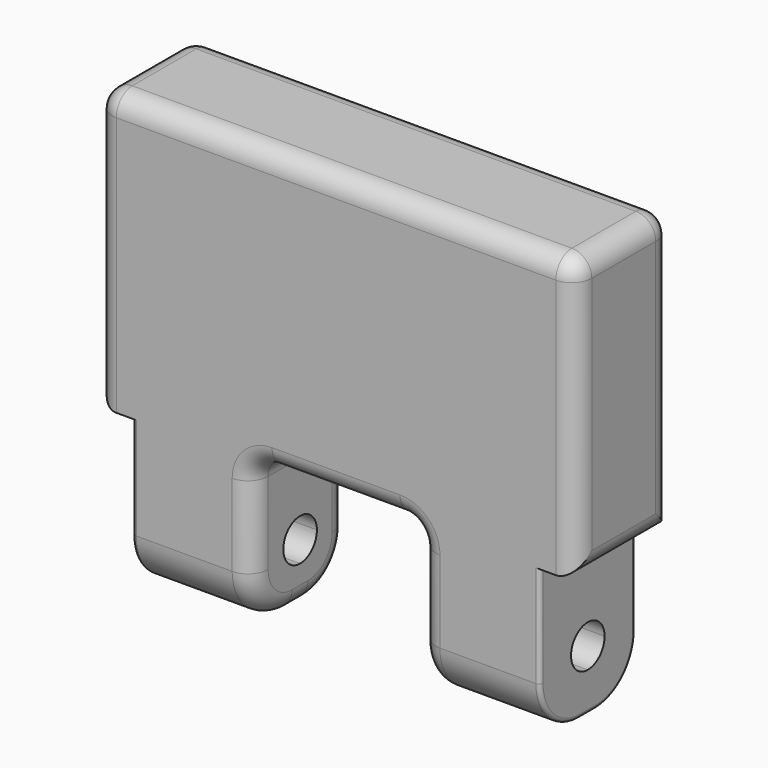
from build123d import *

# Parameters (mm, degrees)
F0_W     = 3
F0_H     = 3.8
F1_DEPTH = 3
F3_DEPTH = 11.101
F4_R     = 1.25
F5_F1_R  = 0.5
F5_F2_R  = 0.5
F6_R     = 0.1


with BuildPart() as f1:
    # F0 (on Front) → F1 (new body)
    with BuildSketch(Plane.XZ):
        Polygon((6, -3.5), (6, 3.5), (0, 3.5), (0, -3.5), (2.1, -3.5), (5.1, -3.5), align=None)
        with Locations((3.6, -5.4)):
            Rectangle(F0_W, F0_H)
        with Locations((-3.6, -5.4)):
            Rectangle(F0_W, F0_H)
        Polygon((0, -3.5), (0, 3.5), (-6, 3.5), (-6, -3.5), (-5.1, -3.5), (-2.1, -3.5), align=None)
    extrude(amount=F1_DEPTH)

    # F2 (on face) → F3 (cut, through all)
    with BuildSketch(Plane.YZ.offset(5.1)):
        with BuildLine():
            ThreePointArc((-1.5, -5.275), (-2.025, -5.8), (-1.5, -6.325))
            Line((-1.5, -6.325), (-1.5, -5.275))
        make_face()
        with BuildLine():
            Line((-1.5, -5.275), (-1.5, -6.325))
            ThreePointArc((-1.5, -6.325), (-1.1287689399, -6.1712310601), (-0.975, -5.8))
            ThreePointArc((-0.975, -5.8), (-1.1287689399, -5.4287689399), (-1.5, -5.275))
        make_face()
    extrude(amount=-F3_DEPTH, mode=Mode.SUBTRACT)

    # F4
    f4_edges = [f1.edges().sort_by_distance(p)[0] for p in [
        (-3.6, -3, -7.3),
        (-3.6, 0, -7.3),
        (3.6, -3, -7.3),
        (3.6, 0, -7.3),
    ]]
    fillet(f4_edges, radius=F4_R)

    # F5: fillet of radius 0.5 on 14 edges, made by hand

    # F5_f1
    f5_f1_edges = [f1.edges().sort_by_distance(p)[0] for p in [
        (-2.1, -1.5, -3.5),
        (2.1, -1.5, -3.5),
    ]]
    fillet(f5_f1_edges, radius=F5_F1_R)

    # F5_f2
    f5_f2_edges = [f1.edges().sort_by_distance(p)[0] for p in [
        (0, 0, -3.5),
        (0, -3, -3.5),
        (-6, -1.5, 3.5),
        (-6, -1.5, -3.5),
        (-6, 0, 0),
        (-6, -3, 0),
        (6, -1.5, -3.5),
        (6, -1.5, 3.5),
        (6, 0, 0),
        (6, -3, 0),
        (0, 0, 3.5),
        (0, -3, 3.5),
        (-1.9535533906, -3, -3.6464466094),
        (1.9535533906, -3, -3.6464466094),
        (-1.9535533906, 0, -3.6464466094),
        (1.9535533906, 0, -3.6464466094),
    ]]
    fillet(f5_f2_edges, radius=F5_F2_R)

    # F6
    f6_edges = [f1.edges().sort_by_distance(p)[0] for p in [
        (-5.1, -2.633883, -6.933883),
        (5.1, -3, -4.775),
    ]]
    fillet(f6_edges, radius=F6_R)


solid = f1.part
